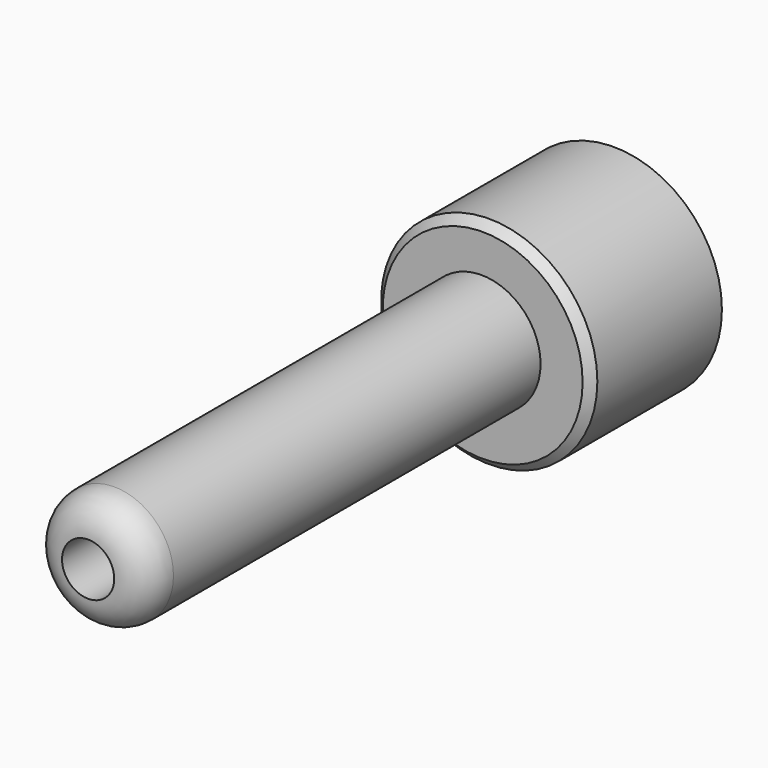
from build123d import *

# Parameters (mm, degrees)
F0_R        = 36.650285017
F1_DEPTH    = 50.8
F2_R        = 16.1794098337
F3_DEPTH    = 127
F5_R        = 28.203657399
F5_R_2      = 16.1794098337
F4_R        = 16.1794098337
F3_FACE_R   = 16.1794098337
F6_DEPTH    = 50.8
F7_DEPTH    = 101.6
F8_DEPTH    = 50.8
F9_DEPTH    = 101.6
F10_DEPTH   = 25.4
F11_R       = 67.0391911282
F9_FACE_R   = 36.650285017
F9_FACE_R_2 = 16.1794098337
F12_DEPTH   = 101.6
F13_R       = 20.32
F14_SIZE    = 5.08


with BuildPart() as f1:
    # F0 (on Front) → F1 (new body)
    with BuildSketch(Plane.XZ):
        Circle(F0_R)
    extrude(amount=F1_DEPTH)

    # F2 (on face) → F3 (join)
    with BuildSketch(Plane.XZ.offset(50.8)):
        Circle(F2_R)
    extrude(amount=F3_DEPTH)

    # F5 (on face) + F4 (on face) + F3_face (on face) → F6 (cut)
    with BuildSketch(Plane.XZ.offset(177.8)):
        Circle(F5_R)
        Circle(F5_R_2, mode=Mode.SUBTRACT)
        Circle(F5_R_2)
    with BuildSketch(Plane.XZ.offset(177.8)):
        Circle(F4_R)
    with BuildSketch(Plane.XZ.offset(177.8)):
        Circle(F3_FACE_R)
    extrude(amount=-F6_DEPTH, mode=Mode.SUBTRACT)

    # F7 (add): faces of the model
    f7_faces = [f1.faces().sort_by_distance(p)[0] for p in [
        (-35.6136584143, -50.8, 0),
        (0, 0, 0),
    ]]
    extrude(f7_faces, amount=F7_DEPTH, dir=(0, -1, 0))

    # F8 (add): faces of the model
    f8_faces = [f1.faces().sort_by_distance(p)[0] for p in [
        (-35.6136584143, -152.4, 0),
        (0, -127, 0),
        (0, 0, 0),
    ]]
    extrude(f8_faces, amount=F8_DEPTH, dir=(0, -1, 0))

    # F9 (add): faces of the model
    f9_faces = [f1.faces().sort_by_distance(p)[0] for p in [
        (-35.6136584143, -203.2, 0),
        (0, 0, 0),
    ]]
    extrude(f9_faces, amount=F9_DEPTH, dir=(0, -1, 0))

    # F10 (add): faces of the model
    f10_faces = [f1.faces().sort_by_distance(p)[0] for p in [
        (0, -177.8, 0),
        (0, 0, 0),
    ]]
    extrude(f10_faces, amount=-F10_DEPTH, dir=(0, -1, 0))

    # F11 (on Front) + F9_face (on face) → F12 (join)
    with BuildSketch(Plane.XZ):
        with Locations((0.7551472518, -1.5102935722)):
            Circle(F11_R)
    with BuildSketch(Plane.XZ.offset(304.8)):
        Circle(F9_FACE_R)
        Circle(F9_FACE_R_2, mode=Mode.SUBTRACT)
    extrude(amount=F12_DEPTH)

    # F13
    f13_edges = [f1.edges().sort_by_distance(p)[0] for p in [
        (-36.650285, -406.4, 0),
    ]]
    fillet(f13_edges, radius=F13_R)

    # F14
    f14_edges = [f1.edges().sort_by_distance(p)[0] for p in [
        (-66.284044, -101.6, -1.510294),
    ]]
    chamfer(f14_edges, length=F14_SIZE)


solid = f1.part
